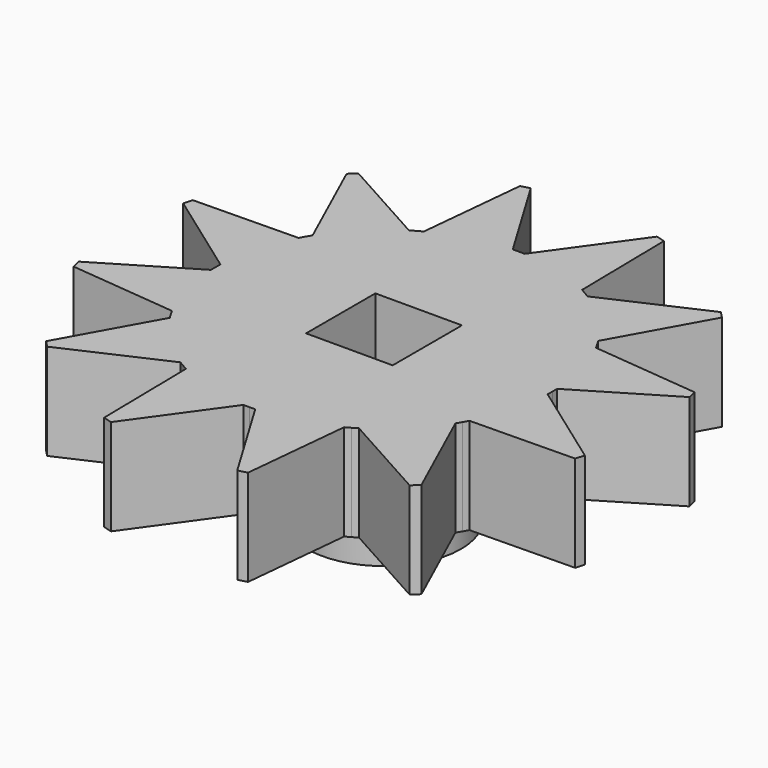
from build123d import *

# Parameters (mm, degrees)
F0_R            = 11
F1_DEPTH        = 4
F3_DEPTH        = 4.001
F3_COPIES_COUNT = 12
F5_R            = 3.2
F6_DEPTH        = 3
F7_W            = 3.6
F7_H            = 3.6
F8_DEPTH        = 7.001


# Not quite as in the source:
# - a pattern or mirror of a feature is missing from the dataset's text; its kind, count and spacing are read off the source's solid


with BuildPart() as f1:
    # F0 (on Top) → F1 (new body)
    with BuildSketch(Plane.XY):
        Circle(F0_R)
    extrude(amount=F1_DEPTH)

    # F2 (on face) → F3 (cut, through all)
    with BuildSketch(Plane.XY.offset(4)):
        with BuildLine():
            Line((0, 11), (0, 7))
            ThreePointArc((0, 7), (0.1221668451, 6.9989338661), (0.2442964769, 6.9957357891))
            Line((0.2442964769, 6.9957357891), (2.8470094961, 10.6251840892))
            ThreePointArc((2.8470094961, 10.6251840892), (1.4357881144, 10.9058934751), (0, 11))
        make_face()
        with BuildLine():
            ThreePointArc((-0.2442964769, 6.9957357891), (-0.1221668451, 6.9989338661), (0, 7))
            Line((0, 7), (0, 11))
            ThreePointArc((0, 11), (-1.2452353514, 10.9292904124), (-2.4744615978, 10.7180707126))
            Line((-2.4744615978, 10.7180707126), (-0.2442964769, 6.9957357891))
        make_face()
    f3 = extrude(amount=-F3_DEPTH, mode=Mode.SUBTRACT)

    # F3_copies: F3 ×12 about axis
    f3_copies_axis = Axis((0, 0, 0), (0, 0, 1))
    for i in range(1, F3_COPIES_COUNT):
        add(f3.rotate(f3_copies_axis, i * 360 / F3_COPIES_COUNT), mode=Mode.SUBTRACT)

    # F5 (on face) → F6 (join)
    with BuildSketch(Plane(origin=(0, 0, 0), x_dir=(1, 0, 0), z_dir=(0, 0, -1))):
        Circle(F5_R)
    extrude(amount=F6_DEPTH)

    # F7 (on face) → F8 (cut, through all)
    with BuildSketch(Plane(origin=(0, 0, -3), x_dir=(1, 0, 0), z_dir=(0, 0, -1))):
        Rectangle(F7_W, F7_H)
    extrude(amount=-F8_DEPTH, mode=Mode.SUBTRACT)


solid = f1.part
